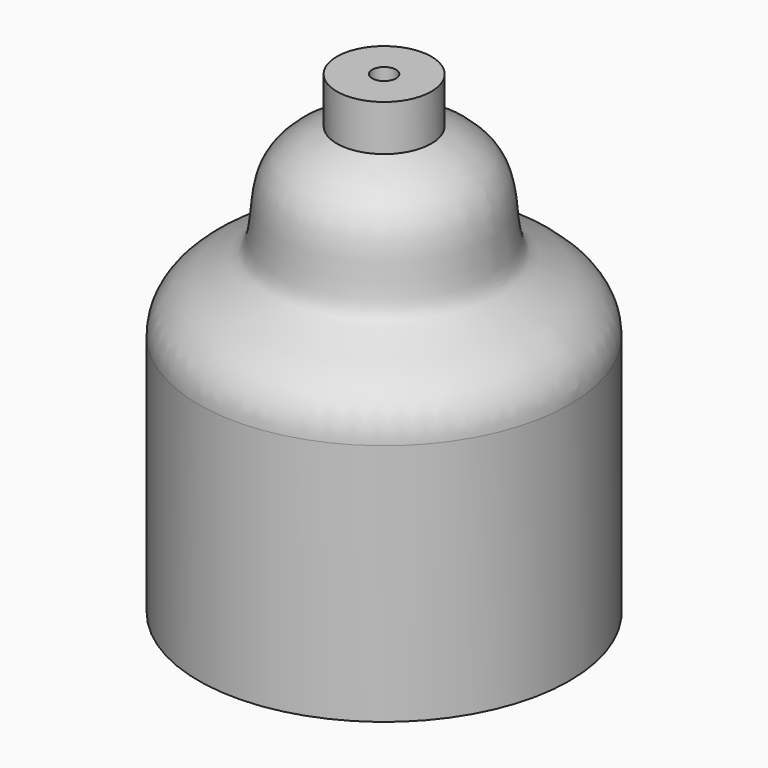
from build123d import *


# Not quite as in the source:
# - ends of sketch curves that miss each other by under 0.0002 mm in the source are joined
# - the dataset's text gives a spline's control points without its knots; the knots are read off the source's solid


with BuildPart() as f1:
    # F0 (on Front) → F1 (revolve)
    with BuildSketch(Plane.XZ):
        with BuildLine():
            Line((50.8, -68.5799818198), (0, -68.5799818198))
            Line((0, -68.5799818198), (0, -74.9299818198))
            Line((0, -74.9299818198), (57.15, -74.9299818198))
            Line((57.15, -74.9299818198), (57.15, 1.6272e-06))
            add(Edge.make_bspline(
                [(57.15, 1.6272e-06), (57.1499999994, 0.7047113918), (57.0598999162, 2.103273417), (56.6515693983, 4.1275628276), (55.9891831776, 6.0294834035), (55.1137080803, 7.7693366077), (54.0770742303, 9.3282529906), (52.5451803539, 11.1692858227), (50.4535495865, 13.0673465504), (47.8521882716, 14.8916410503), (45.252819746, 16.425180894), (42.7316484966, 17.7782729868), (40.3709871587, 19.0241328449), (38.6175601714, 20.0091031011), (37.3964709607, 20.7693815862), (36.5848410934, 21.3222974779), (35.889165019, 21.8521978188), (35.3187701783, 22.3490647419), (34.9484904994, 22.7282804416), (34.7161027204, 23.0004508821), (34.5495368253, 23.2155139733), (34.3902675999, 23.4425507333), (34.1858485185, 23.7641041974), (33.8467702825, 24.3818175191), (33.4109284532, 25.4497498628), (32.9816573877, 27.0498729284), (32.6545525856, 28.932648506), (32.411932376, 31.0443557544), (32.2145322917, 33.3333465292), (32.0061617084, 35.7596304469), (31.7139430509, 38.2985913452), (31.3207822666, 40.5019809383), (30.8480072544, 42.315454933), (30.4671278129, 43.4684021236), (30.0993683091, 44.3969660699), (29.7863286696, 45.0992011119), (29.4431534601, 45.7843141536), (28.9514880524, 46.6664553198), (28.2759351057, 47.710924054), (27.0873755974, 49.2504932123), (25.4420689363, 50.9266202701), (23.3260377998, 52.5809069603), (21.1425673416, 53.9478206558), (18.9367386048, 55.0958122319), (16.73909063, 56.0833338186), (15.292731043, 56.6675944469), (14.5776358142, 56.9480177287), (14.5734167567, 56.9496719276)],
                knots=[1.95e-08, 1.95e-08, 1.95e-08, 1.95e-08, 0.015625, 0.03125, 0.046875, 0.0625, 0.078125, 0.09375, 0.125, 0.15625, 0.1875, 0.21875, 0.25, 0.28125, 0.296875, 0.3125, 0.328125, 0.34375, 0.359375, 0.3671875, 0.375, 0.3828125, 0.390625, 0.40625, 0.4375, 0.46875, 0.5, 0.53125, 0.5625, 0.59375, 0.625, 0.65625, 0.671875, 0.6875, 0.6953125, 0.703125, 0.7109375, 0.71875, 0.734375, 0.75, 0.78125, 0.8125, 0.84375, 0.875, 0.90625, 0.9375, 0.9376854849, 0.9376854849, 0.9376854849, 0.9376854849], degree=3))
            Line((14.5734167567, 56.9496719276), (14.5734162837, 71.0851369262))
            Line((14.5734162837, 71.0851369262), (3.6679329351, 71.0851369262))
            Line((3.6679329351, 71.0851369262), (3.6679329351, 64.7351369262))
            Line((3.6679329351, 64.7351369262), (8.2234162837, 64.7351369262))
            Line((8.2234162837, 64.7351369262), (8.2234162837, 52.5710880756))
            add(Edge.make_bspline(
                [(50.8, 0), (50.8000016062, 10.1355050023), (21.8530368998, 13.6006812311), (29.227455035, 45.4185092323), (14.6406068987, 50.1267635615), (8.2234162837, 52.5710880756)],
                knots=[0, 0, 0, 0, 0.3637012491, 0.7015500616, 1, 1, 1, 1], degree=3))
            Line((50.8, 0), (50.8, -68.5799818198))
        make_face()
    revolve(axis=Axis((0, 0, -71.7549818198), (0, 0, -1)))


solid = f1.part
